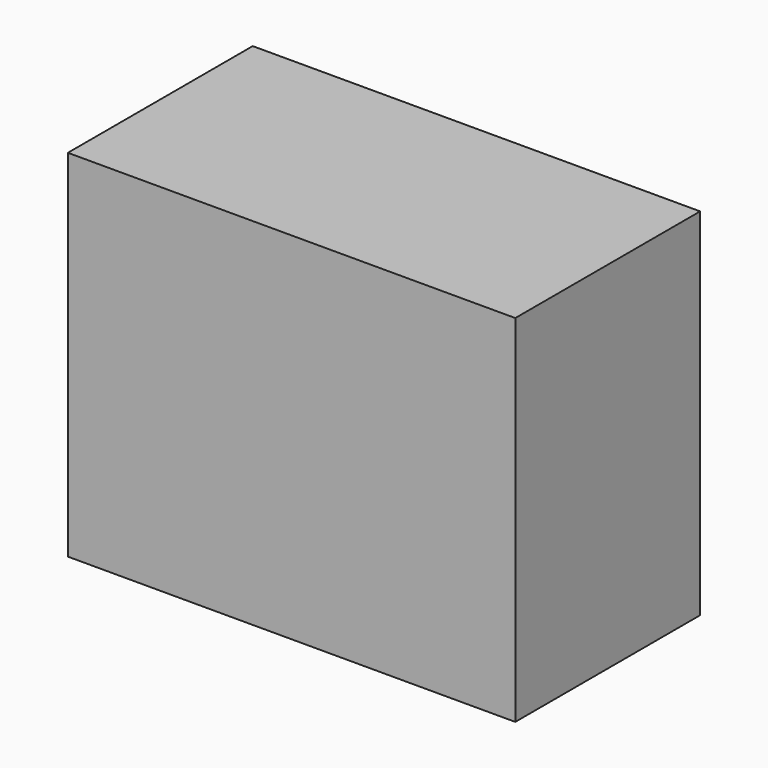
from build123d import *

# Parameters (mm, degrees)
F0_W     = 48.4094880521
F0_H     = 38.4689942002
F1_DEPTH = 25


# Not quite as in the source:
# - a feature of the source that left no trace in its solid (it failed there, or was rolled back) is left out


with BuildPart() as f1:
    # F0 (on Front) → F1 (new body)
    with BuildSketch(Plane.XZ):
        with Locations((-80.1782179624, 56.3604049385)):
            Rectangle(F0_W, F0_H)
    extrude(amount=F1_DEPTH)


solid = f1.part
